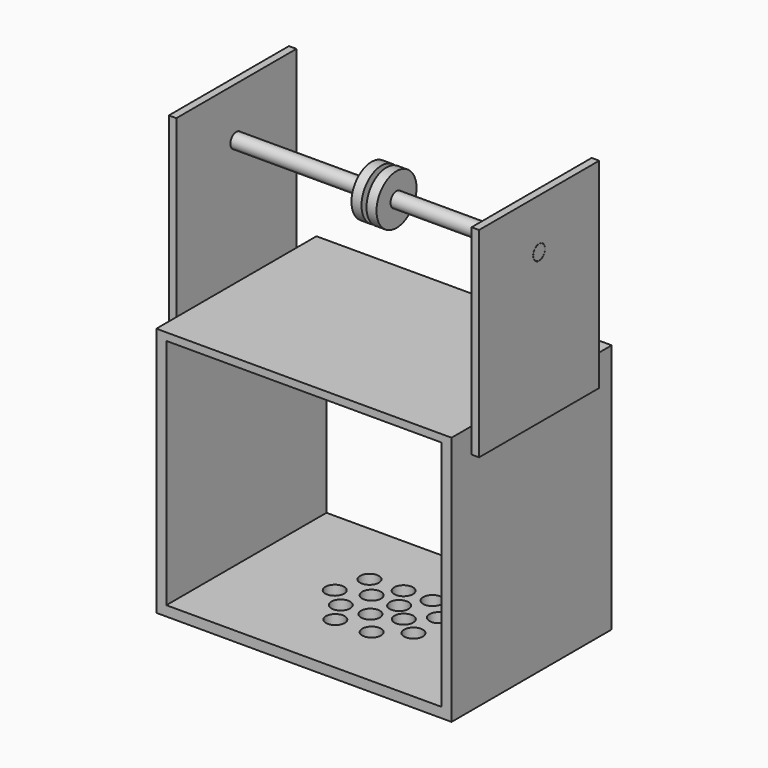
from build123d import *

# Parameters (mm, degrees)
F0_W      = 139.7
F0_H      = 3.81
F0_H_2    = 5.08
F1_DEPTH  = 101.6
F3_DEPTH  = 3.81
F8_R      = 3.81
F9_DEPTH  = 25.4
F10_R     = 3.7465
F11_DEPTH = 157.48
F12_R     = 12.7
F12_R_2   = 3.81
F13_DEPTH = 6.35
F14_T     = -5.08
F15_R     = 4.7625
F16_DEPTH = 5.08
F17_R     = 4.7625
F18_DEPTH = 25.4


# Not quite as in the source:
# - a pattern or mirror of a feature is missing from the dataset's text; its kind, count and spacing are read off the source's solid


with BuildPart() as f1:
    # F0 (on Front) → F1 (new body)
    with BuildSketch(Plane.XZ):
        with Locations((-69.85, -1.905)):
            Rectangle(F0_W, F0_H)
        Polygon((5.08, 0), (0, 0), (0, -3.81), (0, -118.11), (0, -121.92), (0, -127), (5.08, -127), align=None)
        Polygon((-139.7, -3.81), (-139.7, 0), (-144.78, 0), (-144.78, -127), (-139.7, -127), (-139.7, -121.92), (-139.7, -118.11), align=None)
        with Locations((-69.85, -124.46)):
            Rectangle(F0_W, F0_H_2)
    extrude(amount=F1_DEPTH)

    # F2 (on face) → F3 (join)
    with BuildSketch(Plane.YZ.offset(5.08)):
        Polygon((-88.9, 0), (-88.9, -12.7), (-12.7, -12.7), (-12.7, 0), (-12.7, 88.9), (-88.9, 88.9), align=None)
    f3 = extrude(amount=F3_DEPTH)

    # F3_copies: F3 across plane
    add(f3.mirror(Plane(origin=(-69.85, 0, 0), x_dir=(0, 0, -1), z_dir=(-1, 0, 0))))

    # F8 (on face) → F9 (cut)
    with BuildSketch(Plane.YZ.offset(8.89)):
        with Locations((-50.8, 63.5)):
            Circle(F8_R)
    f9 = extrude(amount=-F9_DEPTH, mode=Mode.SUBTRACT)

    # F9_copies: F9 across plane
    add(f9.mirror(Plane(origin=(-69.85, 0, 0), x_dir=(0, 0, -1), z_dir=(-1, 0, 0))), mode=Mode.SUBTRACT)

    # F15 (on face) → F16 (cut, through all)
    with BuildSketch(Plane.XY.offset(-121.92)):
        with Locations((-95.6051437133, -49.8613993831)):
            Circle(F15_R)
        with Locations((-85.808495901, -58.2803937861)):
            Circle(F15_R)
        with Locations((-81.5224657633, -44.0446418892)):
            Circle(F15_R)
        with Locations((-90.7068177886, -33.9418502205)):
            Circle(F15_R)
        with Locations((-74.0219069665, -33.1764875517)):
            Circle(F15_R)
        with Locations((-67.439783776, -44.1977138174)):
            Circle(F15_R)
        with Locations((-71.7258179509, -57.0558102863)):
            Circle(F15_R)
        with Locations((-58.7146475352, -52.1574883987)):
            Circle(F15_R)
        with Locations((-59.7861550696, -32.5641968111)):
            Circle(F15_R)
    extrude(amount=-F16_DEPTH, mode=Mode.SUBTRACT)

    # F17 (on face) → F18 (cut)
    with BuildSketch(Plane.XY.offset(-121.92)):
        with Locations((-48.6777946449, -42.4636480062)):
            Circle(F17_R)
        with Locations((-61.7339971875, -68.7800602236)):
            Circle(F17_R)
        with Locations((-79.6862773542, -69.3920682561)):
            Circle(F17_R)
        with Locations((-48.2490323484, -59.102896601)):
            Circle(F17_R)
    extrude(amount=-F18_DEPTH, mode=Mode.SUBTRACT)


with BuildPart() as f11:
    # F10 (on face) → F11 (new body)
    with BuildSketch(Plane.YZ.offset(8.89)):
        with Locations((-50.8, 63.5)):
            Circle(F10_R)
    extrude(amount=-F11_DEPTH)


with BuildPart() as f13:
    # F12 (on 3pt) → F13 (new body, symmetric)
    with BuildSketch(Plane(origin=(-69.85, 0, 0), x_dir=(0, -1, 0), z_dir=(-1, 0, 0))):
        with Locations((50.8, 63.5)):
            Circle(F12_R)
        with Locations((50.8, 63.5)):
            Circle(F12_R_2, mode=Mode.SUBTRACT)
    extrude(amount=F13_DEPTH, both=True)

    # F14
    f14_openings = [f13.faces().sort_by_distance(p)[0] for p in [
        (-69.85, -38.1, 63.5),
    ]]
    offset(amount=F14_T, openings=f14_openings)


solid = Compound([f1.part, f11.part, f13.part])
